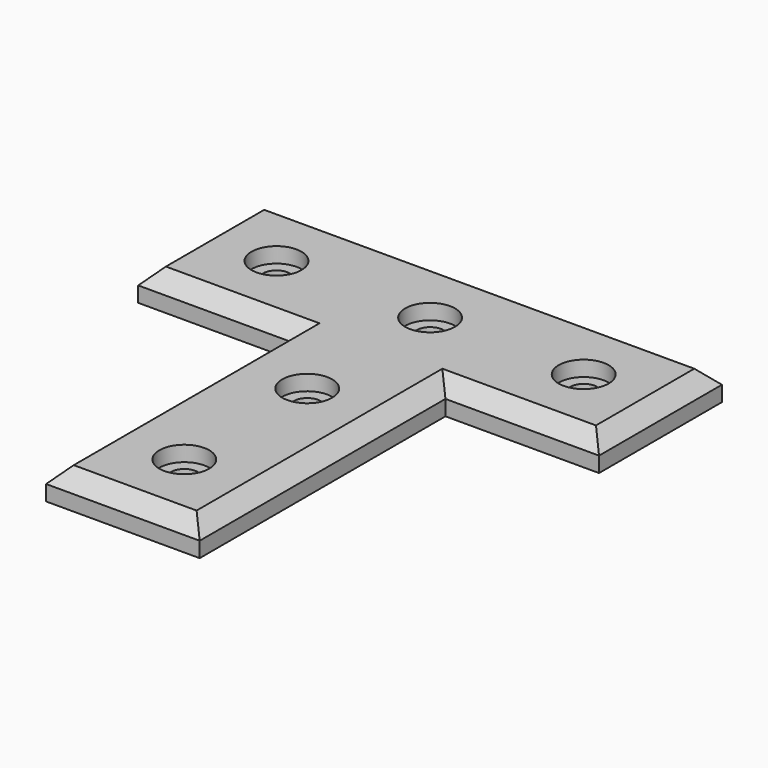
from build123d import *

# Parameters (mm, degrees)
F2_R     = 1.75
F3_DEPTH = 4
F4_SIZE  = 2
F5_R     = 3.25
F5_R_2   = 1.75
F6_DEPTH = 2


with BuildPart() as f3:
    # F2 (on Top) → F3 (new body)
    with BuildSketch(Plane.XY):
        Polygon((-10, -50), (0, -50), (10, -50), (10, -10), (30, -10), (30, 10), (0, 10), (-30, 10), (-30, -10), (-10, -10), align=None)
        with Locations((0, -40)):
            Circle(F2_R, mode=Mode.SUBTRACT)
        with Locations((-20, 0)):
            Circle(F2_R, mode=Mode.SUBTRACT)
        with Locations((0, -20)):
            Circle(F2_R, mode=Mode.SUBTRACT)
        Circle(F2_R, mode=Mode.SUBTRACT)
        with Locations((20, 0)):
            Circle(F2_R, mode=Mode.SUBTRACT)
    extrude(amount=F3_DEPTH)

    # F4
    f4_edges = [f3.edges().sort_by_distance(p)[0] for p in [
        (0, -50, 4),
        (10, -30, 4),
        (20, -10, 4),
        (30, 0, 4),
        (0, 10, 4),
        (-30, 0, 4),
        (-20, -10, 4),
        (-10, -30, 4),
    ]]
    chamfer(f4_edges, length=F4_SIZE)

    # F5 (on face) → F6 (cut)
    with BuildSketch(Plane.XY.offset(4)):
        with Locations((-20, 0)):
            Circle(F5_R)
        with Locations((-20, 0)):
            Circle(F5_R_2, mode=Mode.SUBTRACT)
        Circle(F5_R)
        Circle(F5_R_2, mode=Mode.SUBTRACT)
        with Locations((20, 0)):
            Circle(F5_R)
        with Locations((20, 0)):
            Circle(F5_R_2, mode=Mode.SUBTRACT)
        with Locations((0, -20)):
            Circle(F5_R)
        with Locations((0, -20)):
            Circle(F5_R_2, mode=Mode.SUBTRACT)
        with Locations((0, -40)):
            Circle(F5_R)
        with Locations((0, -40)):
            Circle(F5_R_2, mode=Mode.SUBTRACT)
    extrude(amount=-F6_DEPTH, mode=Mode.SUBTRACT)


solid = f3.part
